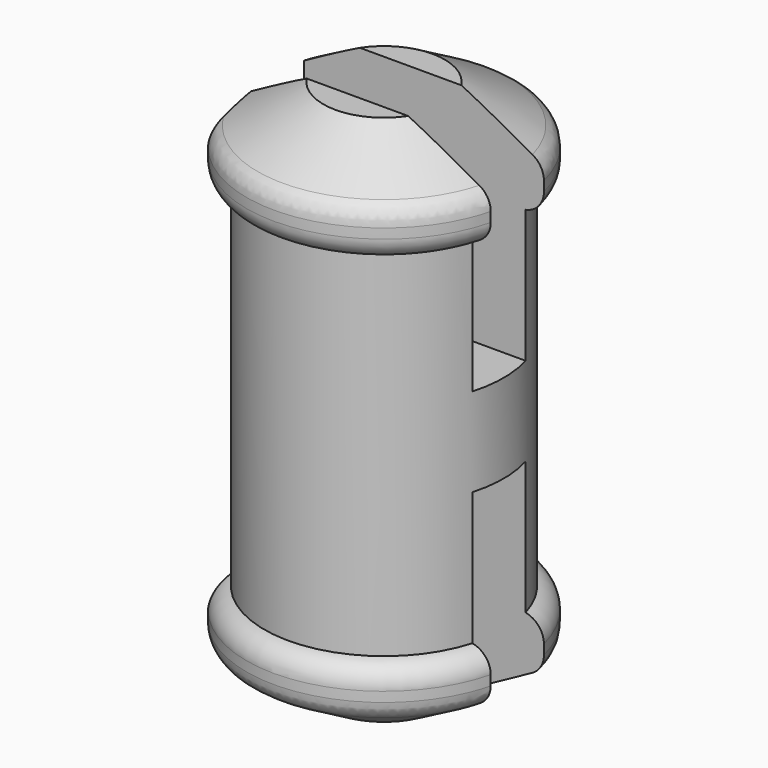
from build123d import *

# Parameters (mm, degrees)
F0_R         = 3.1
F1_DEPTH     = 2
F2_R         = 2.7
F3_DEPTH     = 8
F4_R         = 3.1
F5_DEPTH     = 2
F8_DEPTH     = 5
F10_DEPTH    = 5
F11_C1_SIZE2 = 1
F11_C1_SIZE  = 1.7320508076
F11_C2_SIZE2 = 1
F11_C2_SIZE  = 1.7320508076
F12_C1_SIZE2 = 1
F12_C1_SIZE  = 1.7320508076
F12_C2_SIZE2 = 1
F12_C2_SIZE  = 1.7320508076
F13_R        = 0.5
F15_DEPTH    = 25


# Not quite as in the source:
# - a fillet or chamfer that OpenCascade refuses, or shapes differently, is made with other operations: its cross-section is extruded or revolved along the edge and cut away or added


with BuildPart() as f1:
    # F0 (on Top) → F1 (new body)
    with BuildSketch(Plane.XY):
        Circle(F0_R)
    extrude(amount=F1_DEPTH)

    # F2 (on face) → F3 (join)
    with BuildSketch(Plane.XY.offset(2)):
        Circle(F2_R)
    extrude(amount=F3_DEPTH)

    # F4 (on face) → F5 (join)
    with BuildSketch(Plane.XY.offset(10)):
        Circle(F4_R)
    extrude(amount=F5_DEPTH)

    # F6: fillet of radius 0.5 on 2 edges, made by hand

    # F6_s1 → F6_t2 (revolve, cut)
    with BuildSketch(Plane.XZ):
        with BuildLine():
            ThreePointArc((2.7, 2), (2.9872983346, 1.8263298175), (3.1, 1.5101020514))
            Line((3.1, 1.5101020514), (3.1, 2))
            Line((3.1, 2), (2.7, 2))
        make_face()
    revolve(axis=Axis((0, 0, 2), (0, 0, 1)), mode=Mode.SUBTRACT)

    # F6_s3 → F6_t4 (revolve, cut)
    with BuildSketch(Plane.XZ):
        with BuildLine():
            ThreePointArc((3.1, 10.4898979486), (2.9872983346, 10.1736701825), (2.7, 10))
            Line((2.7, 10), (3.1, 10))
            Line((3.1, 10), (3.1, 10.4898979486))
        make_face()
    revolve(axis=Axis((0, 0, 10), (0, 0, 1)), mode=Mode.SUBTRACT)

    # F7 (on face) → F8 (cut)
    with BuildSketch(Plane(origin=(0, 0, 0), x_dir=(1, 0, 0), z_dir=(0, 0, -1))):
        with BuildLine():
            ThreePointArc((-3.0079062485, 0.75), (-3.1083608316, 0), (-3.0079062485, -0.75))
            Line((-3.0079062485, -0.75), (3.0079062485, -0.75))
            ThreePointArc((3.0079062485, -0.75), (3.1083608316, 0), (3.0079062485, 0.75))
            Line((3.0079062485, 0.75), (-3.0079062485, 0.75))
        make_face()
    extrude(amount=-F8_DEPTH, mode=Mode.SUBTRACT)

    # F9 (on face) → F10 (cut)
    with BuildSketch(Plane.XY.offset(12)):
        with BuildLine():
            ThreePointArc((-3.0079062485, 0.75), (-3.1083608316, 0), (-3.0079062485, -0.75))
            Line((-3.0079062485, -0.75), (3.0079062485, -0.75))
            ThreePointArc((3.0079062485, -0.75), (3.1083608316, 0), (3.0079062485, 0.75))
            Line((3.0079062485, 0.75), (-3.0079062485, 0.75))
        make_face()
    extrude(amount=-F10_DEPTH, mode=Mode.SUBTRACT)

    # F11: chamfer of 1 x 1.7320508076 on 2 edges, made by hand

    # F11_c1
    f11_c1_edges = [f1.edges().sort_by_distance(p)[0] for p in [
        (0, 3.1, 0),
    ]]
    f11_c1_side = f1.faces().sort_by_distance((0, 3.08, 0))[0]
    chamfer(f11_c1_edges, length=F11_C1_SIZE, length2=F11_C1_SIZE2, reference=f11_c1_side)

    # F11_c2
    f11_c2_edges = [f1.edges().sort_by_distance(p)[0] for p in [
        (0, -3.1, 0),
    ]]
    f11_c2_side = f1.faces().sort_by_distance((0, -3.08, 0))[0]
    chamfer(f11_c2_edges, length=F11_C2_SIZE, length2=F11_C2_SIZE2, reference=f11_c2_side)

    # F12: chamfer of 1 x 1.7320508076 on 2 edges, made by hand

    # F12_c1
    f12_c1_edges = [f1.edges().sort_by_distance(p)[0] for p in [
        (0, -3.1, 12),
    ]]
    f12_c1_side = f1.faces().sort_by_distance((0, -3.08, 12))[0]
    chamfer(f12_c1_edges, length=F12_C1_SIZE, length2=F12_C1_SIZE2, reference=f12_c1_side)

    # F12_c2
    f12_c2_edges = [f1.edges().sort_by_distance(p)[0] for p in [
        (0, 3.1, 12),
    ]]
    f12_c2_side = f1.faces().sort_by_distance((0, 3.08, 12))[0]
    chamfer(f12_c2_edges, length=F12_C2_SIZE, length2=F12_C2_SIZE2, reference=f12_c2_side)

    # F13
    f13_edges = [f1.edges().sort_by_distance(p)[0] for p in [
        (0, -3.1, 11),
        (0, 3.1, 11),
        (0, -3.1, 1),
        (0, 3.1, 1),
    ]]
    fillet(f13_edges, radius=F13_R)

    # F14 (on face) → F15 (cut)
    with BuildSketch(Plane.XY.offset(12)):
        with BuildLine():
            Line((-2.4, -1.962141687), (-2.4, 1.962141687))
            ThreePointArc((-2.4, 1.962141687), (-3.1, 0), (-2.4, -1.962141687))
        make_face()
    extrude(amount=-F15_DEPTH, mode=Mode.SUBTRACT)


solid = f1.part
